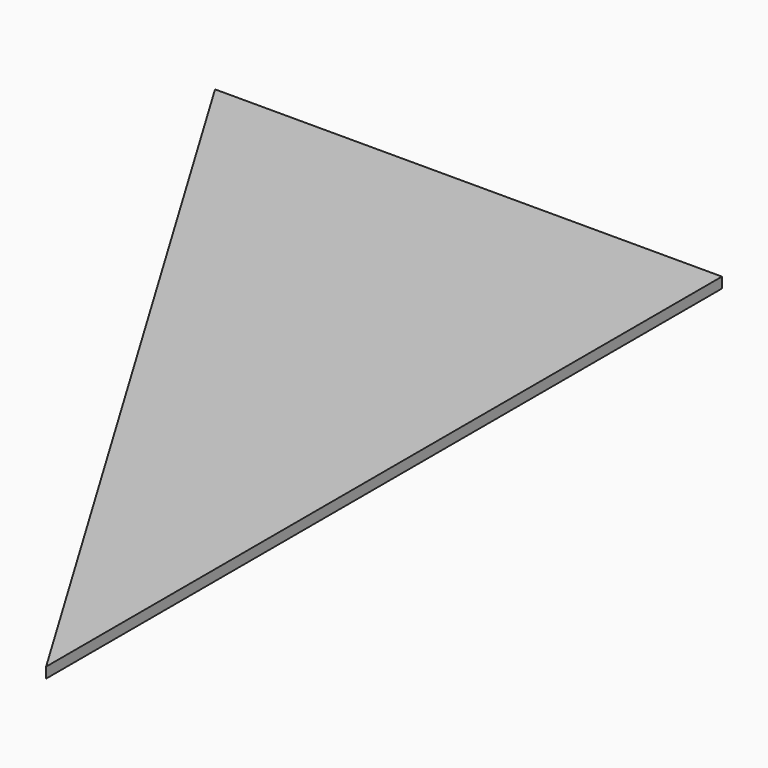
from build123d import *

# Parameters (mm, degrees)
F1_DEPTH = 3.175


# Not quite as in the source:
# - a length typed as a fraction of an inch, garbled in the dataset ("3 / 203.2 mm" for 3/8 in), is restored


with BuildPart() as f1:
    # F0 (on Top) → F1 (new body)
    with BuildSketch(Plane.XY):
        Polygon((0, -254), (0, 0), (-152.4, 0), align=None)
    extrude(amount=F1_DEPTH)


solid = f1.part
